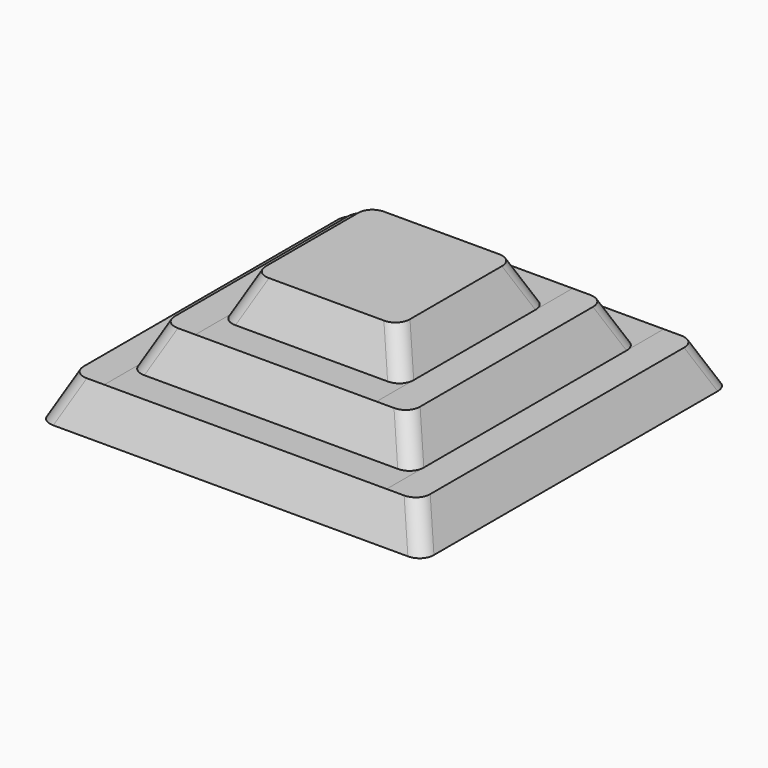
from build123d import *

# Parameters (mm, degrees)
F1_DEPTH = 487.68
F3_DEPTH = 543.56
F4_R     = 25.4


# Not quite as in the source:
# - ends of sketch curves that miss each other by under 0.0002 mm in the source are joined


with BuildPart() as f1:
    # F0 (on Front) → F1 (new body, symmetric)
    with BuildSketch(Plane.XZ):
        Polygon((-83.2644920098, 41.3985210439), (60.6460442831, 41.3985210439), (60.6460442831, 104.8985210439), (-53.6539557169, 104.8985210439), align=None)
        Polygon((60.6460442831, 104.8985210439), (60.6460442831, 41.3985210439), (204.5565805759, 41.3985210439), (174.9460442831, 104.8985210439), align=None)
        Polygon((60.6460442831, 41.3985210439), (60.6460442831, -22.1014789561), (284.9671168688, -22.1014789561), (255.3565805759, 41.3985210439), (204.5565805759, 41.3985210439), align=None)
        Polygon((-163.6750283026, -22.1014789561), (60.6460442831, -22.1014789561), (60.6460442831, 41.3985210439), (-83.2644920098, 41.3985210439), (-134.0644920098, 41.3985210439), align=None)
        Polygon((-244.0855645955, -85.6014789561), (60.6460442831, -85.6014789561), (60.6460442831, -22.1014789561), (-163.6750283026, -22.1014789561), (-214.4750283026, -22.1014789561), align=None)
        Polygon((60.6460442831, -22.1014789561), (60.6460442831, -85.6014789561), (365.3776531616, -85.6014789561), (335.7671168688, -22.1014789561), (284.9671168688, -22.1014789561), align=None)
    extrude(amount=F1_DEPTH, both=True)

    # F2 (on Right) → F3 (cut, symmetric)
    with BuildSketch(Plane.YZ):
        Polygon((-396.5238630772, -85.6014788151), (-294.9238630772, -85.6014788151), (-265.3133267843, -22.1014788151), (-214.5133267843, -22.1014788151), (-184.9027904915, 41.3985211849), (-134.1027904915, 41.3985211849), (-104.4922541986, 104.8985211849), (-180.6922541986, 104.8985211849), (-487.68, 104.8985210439), (-487.68, -85.6014789561), align=None)
        Polygon((284.928818387, -22.1014788151), (314.5393546799, -85.6014788151), (487.68, -85.6014789561), (487.68, 104.8985210439), (124.1077458014, 104.8985210439), (153.7182820942, 41.3985211849), (204.5182820942, 41.3985211849), (234.128818387, -22.1014788151), align=None)
    extrude(amount=F3_DEPTH, both=True, mode=Mode.SUBTRACT)

    # F4
    f4_edges = [f1.edges().sort_by_distance(p)[0] for p in [
        (-68.459224, 138.913014, 73.148521),
        (-148.86976, 219.32355, 9.648521),
        (-229.280296, 299.734087, -53.851479),
        (350.572385, 299.734087, -53.851479),
        (270.161849, 219.32355, 9.648521),
        (189.751312, 138.913014, 73.148521),
        (350.572385, -280.118595, -53.851479),
        (270.161849, -199.708059, 9.648521),
        (189.751312, -119.297522, 73.148521),
        (-229.280296, -280.118595, -53.851479),
        (-148.86976, -199.708059, 9.648521),
        (-68.459224, -119.297522, 73.148521),
    ]]
    fillet(f4_edges, radius=F4_R)


solid = f1.part
